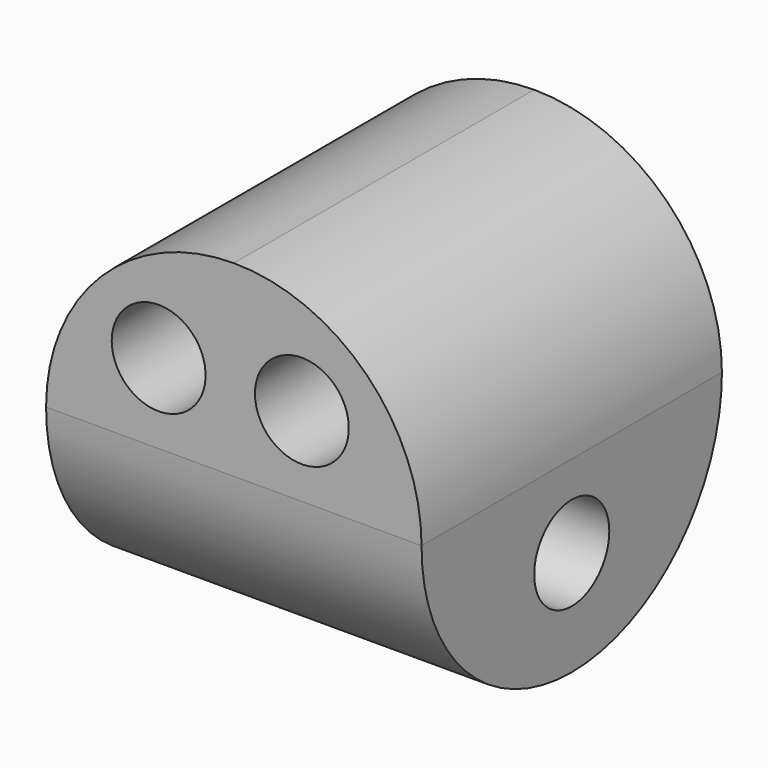
from build123d import *

# Parameters (mm, degrees)
F0_W     = 20
F0_H     = 20
F1_DEPTH = 20
F2_R     = 9.99999
F5_D     = 5
F6_D     = 5


# Not quite as in the source:
# - a fillet or chamfer is up to 0.001 mm smaller than in the source, because OpenCascade refuses the exact size


with BuildPart() as f1:
    # F0 (on Top) → F1 (new body)
    with BuildSketch(Plane.XY):
        Rectangle(F0_W, F0_H)
    extrude(amount=F1_DEPTH)

    # F2 (radius 10 in the source; OpenCascade refuses exactly that, so slightly less here)
    f2_edges = [f1.edges().sort_by_distance(p)[0] for p in [
        (10, 0, 20),
        (-10, 0, 20),
        (0, -10, 0),
        (0, 10, 0),
    ]]
    fillet(f2_edges, radius=F2_R)

    # F5 (through all)
    with Locations(Plane(origin=(-10, 0, 0), x_dir=(0, -1, 0), z_dir=(-1, 0, 0))):
        with Locations((0, 5.5952616967)):
            Hole(F5_D / 2)

    # F6 (through all)
    with Locations(Plane.XZ.offset(10)):
        with Locations((-4.0043536574, 14.245916158), (3.62556451, 14.245916158)):
            Hole(F6_D / 2)


solid = f1.part
